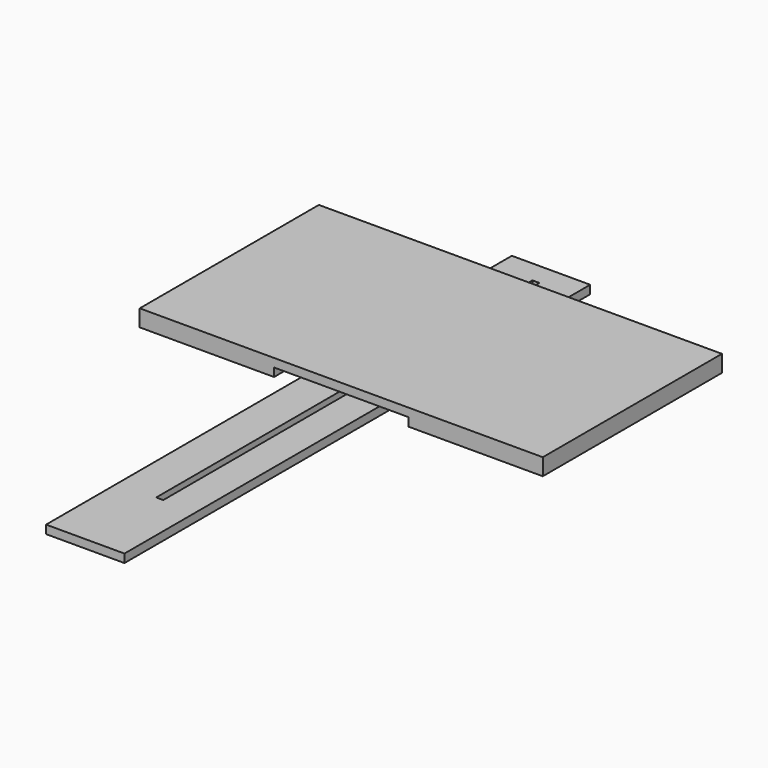
from build123d import *

# Parameters (mm, degrees)
F0_W     = 457.2
F0_H     = 254
F1_DEPTH = 9.525
F2_W     = 152.4
F2_H     = 254
F3_DEPTH = 9.525
F4_W     = 88.9
F4_H     = 660.3725897312
F5_DEPTH = 9.525
F6_W     = 8
F6_H     = 533.3725897312
F7_DEPTH = 9.525


# Not quite as in the source:
# - a length typed as a fraction of an inch, garbled in the dataset ("3 / 203.2 mm" for 3/8 in), is restored


with BuildPart() as f1:
    # F0 (on Top) → F1 (new body)
    with BuildSketch(Plane.XY):
        with Locations((-2.023909241, -29.7276111473)):
            Rectangle(F0_W, F0_H)
    extrude(amount=F1_DEPTH)

    # F2 (on face) → F3 (join)
    with BuildSketch(Plane(origin=(0, 0, 0), x_dir=(1, 0, 0), z_dir=(0, 0, -1))):
        with Locations((-154.423909241, 29.7276111473)):
            Rectangle(F2_W, F2_H)
        with Locations((150.376090759, 29.7276111473)):
            Rectangle(F2_W, F2_H)
    extrude(amount=F3_DEPTH)


with BuildPart() as f5:
    # F4 (on face) → F5 (new body)
    with BuildSketch(Plane(origin=(0, 0, 0), x_dir=(1, 0, 0), z_dir=(0, 0, -1))):
        with Locations((-3.192269256, 188.0340722744)):
            Rectangle(F4_W, F4_H)
    extrude(amount=F5_DEPTH)

    # F6 (on face) → F7 (cut, through all)
    with BuildSketch(Plane(origin=(0, 0, -9.525), x_dir=(1, 0, 0), z_dir=(0, 0, -1))):
        with Locations((0, 149.9340722744)):
            Rectangle(F6_W, F6_H)
    extrude(amount=-F7_DEPTH, mode=Mode.SUBTRACT)


solid = Compound([f1.part, f5.part])
